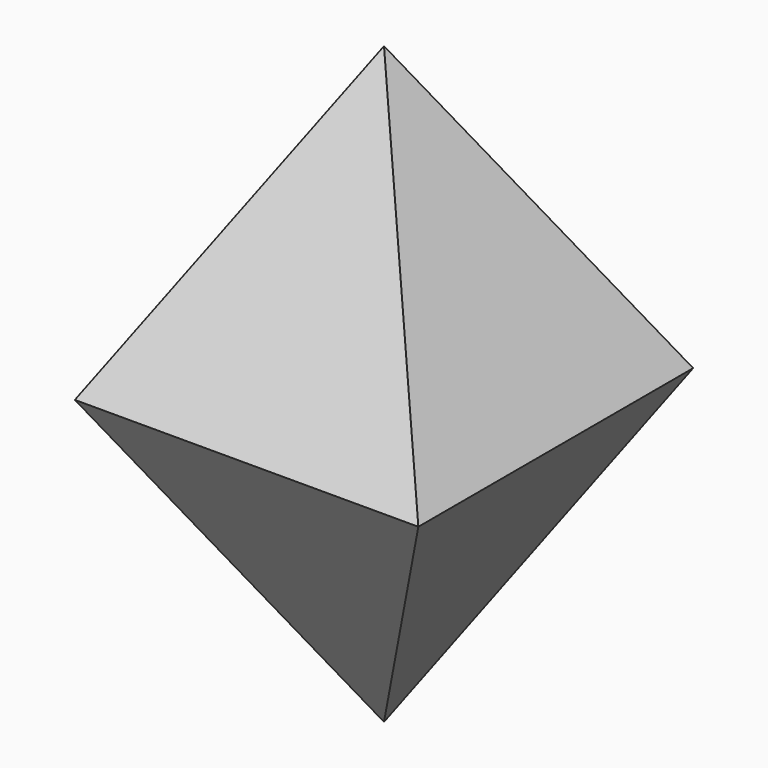
from build123d import *

# Parameters (mm, degrees)
F0_W      = 50.8
F0_H      = 50.8
F1_DEPTH  = 58.166
F1_TAPER  = 30
F1_FACE_W = 50.8
F1_FACE_H = 50.8


# Not quite as in the source:
# - an extrude whose draft closes it to a point is written as a loft to that point


with BuildPart() as f1:
    # F0 (on Top) → F1 (new body)
    with BuildSketch(Plane.XY):
        Rectangle(F0_W, F0_H)
    extrude(amount=F1_DEPTH, taper=F1_TAPER)

    # F1_face (on face) → F2 section 0
    with BuildSketch(Plane(origin=(0, 0, 0), x_dir=(1, 0, 0), z_dir=(0, 0, -1)), mode=Mode.PRIVATE) as f2_s0:
        Rectangle(F1_FACE_W, F1_FACE_H)
    loft([f2_s0.sketch, Vertex(0, 0, -43.9940905122)], ruled=True)


solid = f1.part
